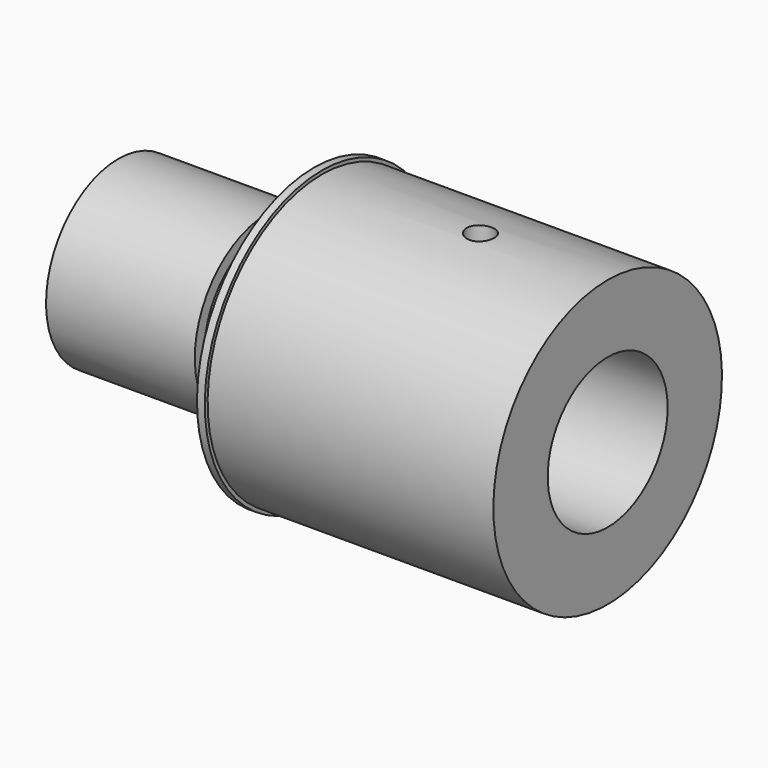
from build123d import *

# Parameters (mm, degrees)
F3_D           = 1
F3_DEPTH       = 65
F3_CBORE_D     = 38.3
F3_CBORE_DEPTH = 65
F3_TIP         = 0.3004303095
F5_D           = 7
F5_DEPTH       = 37.401


# Not quite as in the source:
# - a feature names something its author has since deleted; it is built from what else it names


with BuildPart() as f1:
    # F0 (on Front) → F1 (revolve)
    with BuildSketch(Plane.XZ):
        Polygon((0, 23.1), (0, 0), (125, 0), (125, 36.5), (52, 36.5), (52, 37.4), (50, 37.4), (50, 36.5), (50, 20.1), (38, 20.1), (38, 23.1), align=None)
    revolve(axis=Axis((62.5, 0, 0), (-1, 0, 0)))

    # F3
    with Locations(Plane.YZ.offset(125)):
        with Locations((0, 0)):
            CounterBoreHole(F3_D / 2, F3_CBORE_D / 2, F3_CBORE_DEPTH, depth=F3_DEPTH)
            with Locations((0, 0, -(F3_DEPTH + F3_TIP / 2))):  # 118° drill point
                Cone(0, F3_D / 2, F3_TIP, mode=Mode.SUBTRACT)

    # F5 (through all, one way)
    with BuildSketch(Plane(origin=(0, 0, 0), x_dir=(1, 0, 0), z_dir=(0, 0, -1))):
        with Locations((92.5, 0)):
            Circle(F5_D / 2)
    extrude(amount=-F5_DEPTH, mode=Mode.SUBTRACT)


solid = f1.part
